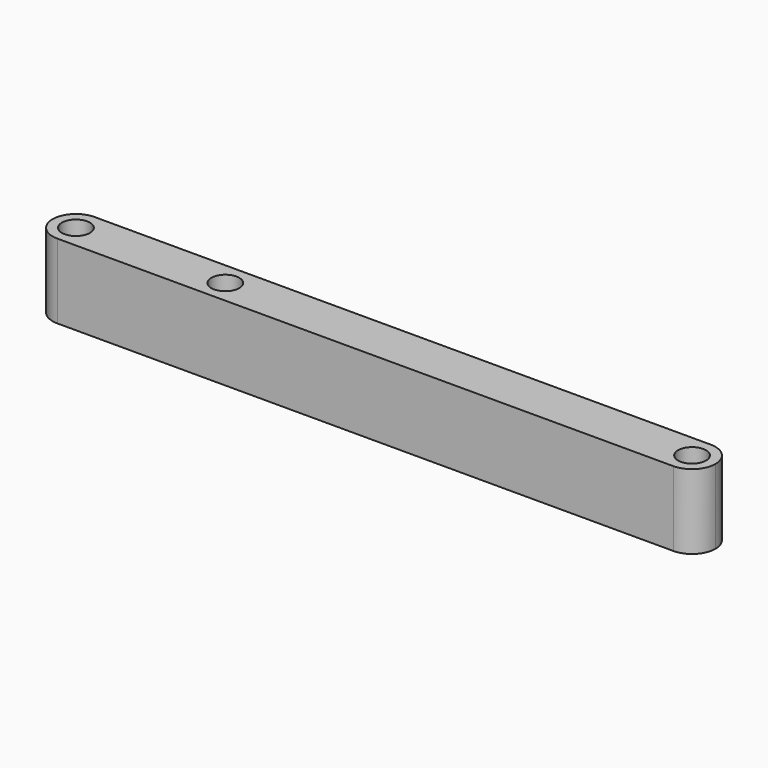
from build123d import *

# Parameters (mm, degrees)
F0_W     = 225.425
F0_H     = 15.875
F1_DEPTH = 25.4
F3_D     = 9.525
F4_R     = 7.93749


# Not quite as in the source:
# - a fillet or chamfer is up to 0.001 mm smaller than in the source, because OpenCascade refuses the exact size


with BuildPart() as f1:
    # F0 (on Top) → F1 (new body)
    with BuildSketch(Plane.XY):
        Rectangle(F0_W, F0_H)
    extrude(amount=F1_DEPTH)

    # F3 (through all)
    with Locations(Plane.XY.offset(25.4)):
        with Locations((104.775, 0), (-104.775, 0), (-53.975, 0)):
            Hole(F3_D / 2)

    # F4 (radius 7.9375 in the source; OpenCascade refuses exactly that, so slightly less here)
    f4_edges = [f1.edges().sort_by_distance(p)[0] for p in [
        (-112.7125, -7.9375, 12.7),
        (112.7125, -7.9375, 12.7),
        (112.7125, 7.9375, 12.7),
        (-112.7125, 7.9375, 12.7),
    ]]
    fillet(f4_edges, radius=F4_R)


solid = f1.part
